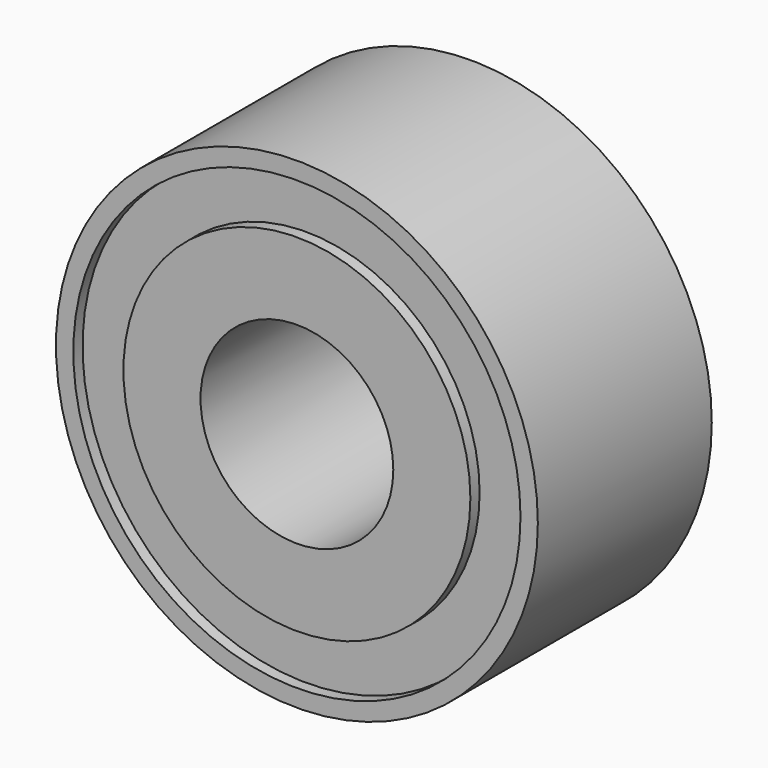
from build123d import *

# Parameters (mm, degrees)
F0_R     = 7.9375
F0_R_2   = 5.08
F1_DEPTH = 3.5814
F2_R     = 7.366
F2_R_2   = 5.715
F3_DEPTH = 0.381
F4_R     = 5.08
F4_R_2   = 3.175
F5_DEPTH = 3.5814


# Not quite as in the source:
# - a pattern or mirror of a feature is missing from the dataset's text; its kind, count and spacing are read off the source's solid


with BuildPart() as f1:
    # F0 (on Front) → F1 (new body, symmetric)
    with BuildSketch(Plane.XZ):
        Circle(F0_R)
        Circle(F0_R_2, mode=Mode.SUBTRACT)
    extrude(amount=F1_DEPTH, both=True)

    # F2 (on face) → F3 (cut)
    with BuildSketch(Plane.XZ.offset(3.5814)):
        Circle(F2_R)
        Circle(F2_R_2, mode=Mode.SUBTRACT)
    f3 = extrude(amount=-F3_DEPTH, mode=Mode.SUBTRACT)

    # F3_copies: F3 across plane
    add(f3.mirror(Plane.ZX), mode=Mode.SUBTRACT)

    # F4 (on Front) → F5 (join, symmetric)
    with BuildSketch(Plane.XZ):
        Circle(F4_R)
        Circle(F4_R_2, mode=Mode.SUBTRACT)
    extrude(amount=F5_DEPTH, both=True)


solid = f1.part
